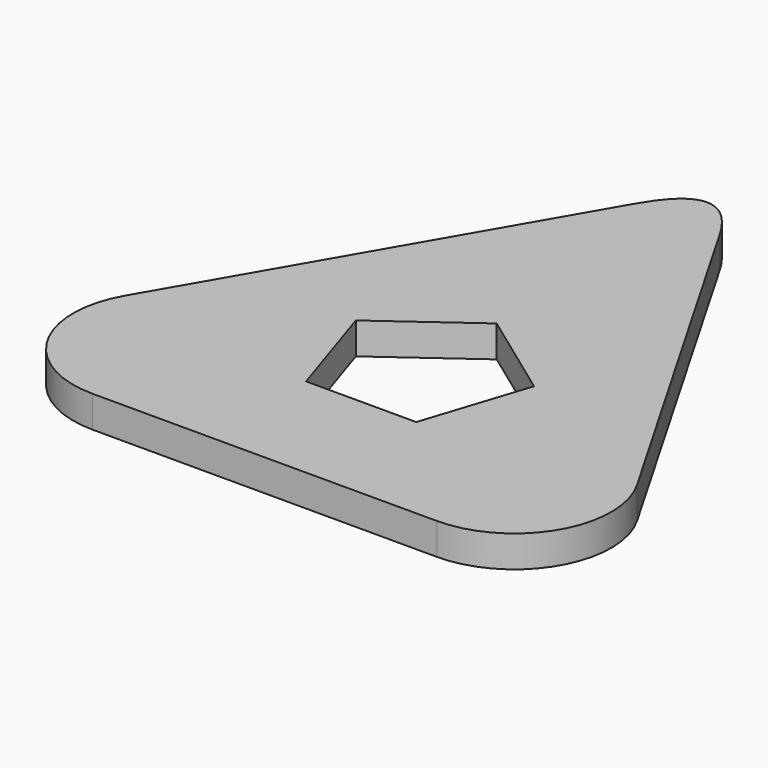
from build123d import *

# Parameters (mm, degrees)
F1_DEPTH    = 1.65862
F2_T1_DEPTH = 23.6556652561
F3_R        = 5.08
F4_R        = 5.08
F6_DEPTH    = 25.4


# Not quite as in the source:
# - a fillet or chamfer that OpenCascade refuses, or shapes differently, is made with other operations: its cross-section is extruded or revolved along the edge and cut away or added


with BuildPart() as f1:
    # F0 (on Top) → F1 (new body)
    with BuildSketch(Plane.XY):
        Polygon((17.8223861725, -10.2897594543), (0, 20.5795189086), (-17.8223861725, -10.2897594543), align=None)
    extrude(amount=F1_DEPTH)

    # F2: fillet of radius 2.54 on 1 edges, made by hand

    # F2_s2 → F2_t1 (cut)
    with BuildSketch(Plane.XY.offset(-10.9985226281)):
        with BuildLine():
            add(Edge.make_bspline(
                [(2.1997045256, 16.7695189086), (0, 20.5795189086), (-2.1997045256, 16.7695189086)],
                knots=[0, 0, 0, 1, 1, 1], degree=2, weights=[1, 1, 1]))
            Line((-2.1997045256, 16.7695189086), (0, 20.5795189086))
            Line((0, 20.5795189086), (2.1997045256, 16.7695189086))
        make_face()
    extrude(amount=F2_T1_DEPTH, mode=Mode.SUBTRACT)

    # F3
    f3_edges = [f1.edges().sort_by_distance(p)[0] for p in [
        (-17.822386, -10.289759, 0.82931),
    ]]
    fillet(f3_edges, radius=F3_R)

    # F4
    f4_edges = [f1.edges().sort_by_distance(p)[0] for p in [
        (17.822386, -10.289759, 0.82931),
    ]]
    fillet(f4_edges, radius=F4_R)

    # F5 (on face) → F6 (cut)
    with BuildSketch(Plane.XY.offset(1.65862)):
        Polygon((4.6700308471, 1.5173850042), (0, 4.9103610218), (-4.6700308471, 1.5173850042), (-2.886237792, -3.9725655151), (2.886237792, -3.9725655151), align=None)
    extrude(amount=-F6_DEPTH, mode=Mode.SUBTRACT)


solid = f1.part
